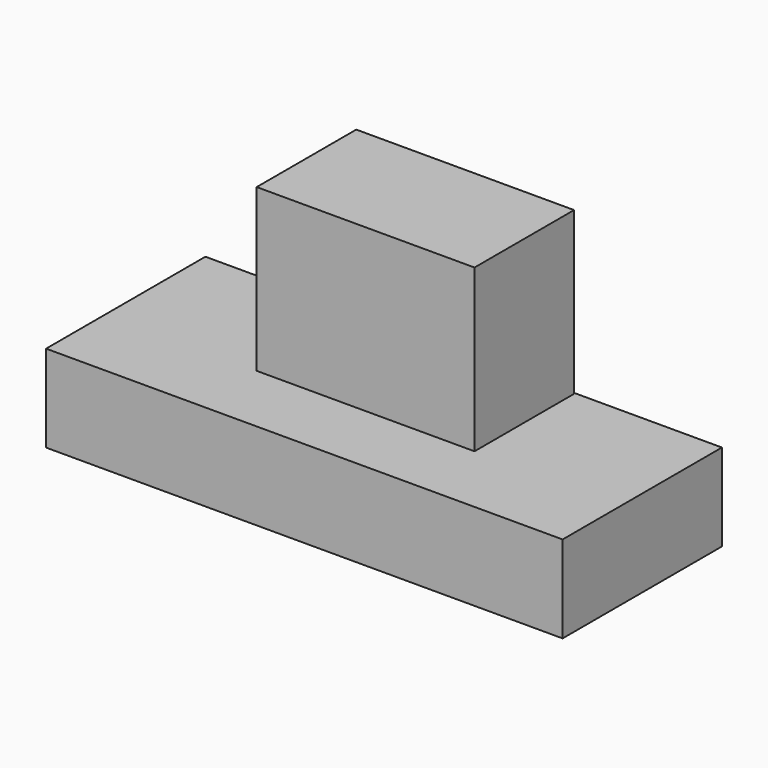
from build123d import *

# Parameters (mm, degrees)
F0_W     = 131.7625
F0_H     = 50.8
F1_DEPTH = 22.225
F3_W     = 55.5625
F3_H     = 31.75
F4_DEPTH = 41.275


# Not quite as in the source:
# - a length typed as a fraction of an inch, garbled in the dataset ("3 / 203.2 mm" for 3/8 in), is restored


with BuildPart() as f1:
    # F0 (on Top) → F1 (new body)
    with BuildSketch(Plane.XY):
        with Locations((-36.3871701598, -7.6868437886)):
            Rectangle(F0_W, F0_H)
    extrude(amount=F1_DEPTH)

    # F3 (on face) → F4 (join)
    with BuildSketch(Plane.XY.offset(22.225)):
        with Locations((-35.7438139617, 1.5146372089)):
            Rectangle(F3_W, F3_H)
    extrude(amount=F4_DEPTH)


solid = f1.part
